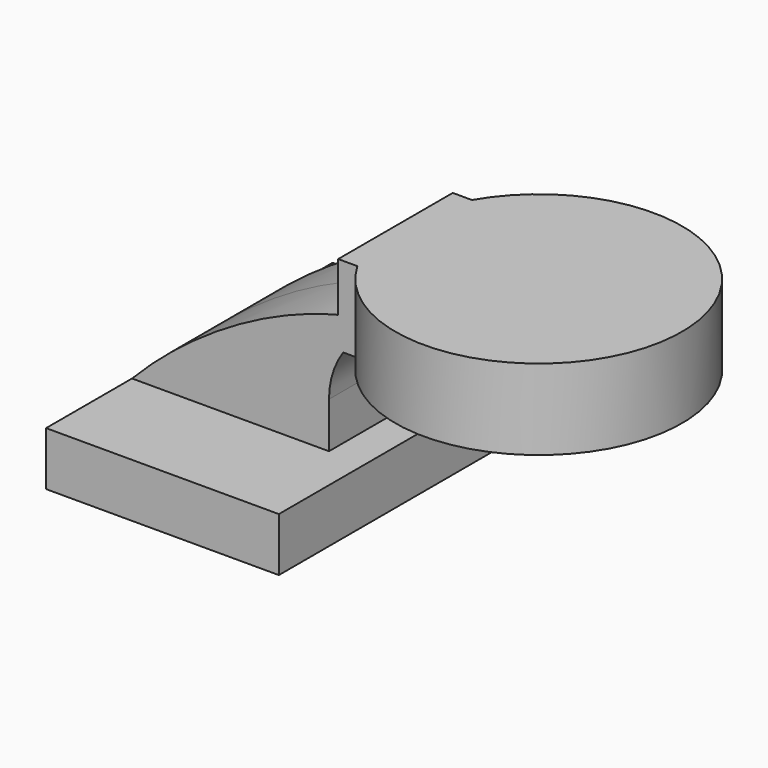
from build123d import *

# Parameters (mm, degrees)
F1_DEPTH = 63.5
F2_DEPTH = 25.4
F3_DEPTH = 25.4


# Not quite as in the source:
# - a feature names something its author has since deleted; it is built from what else it names


with BuildPart() as f1:
    # F0 (on Front) → F1 (new body, symmetric)
    with BuildSketch(Plane.XZ):
        Polygon((28.5749990565, 9.525), (-41.275, 9.525), (-41.275, -9.525), (41.275, -9.525), (41.275, 9.525), align=None)
    extrude(amount=F1_DEPTH, both=True)

    # F0 (on Front) → F2 (join, symmetric)
    with BuildSketch(Plane.XZ):
        with BuildLine():
            add(Edge.make_bspline(
                [(-41.275, 9.525), (-23.8584346144, 27.5869780948), (3.0069667421, 45.9865968148), (31.8262, 53.1677247911)],
                knots=[0, 0, 0, 0, 84.5177049164, 84.5177049164, 84.5177049164, 84.5177049164], degree=3))
            Line((-41.275, 9.525), (28.5749990565, 9.525))
            Line((28.5749990565, 9.525), (28.5749990565, 25.7647229111))
            ThreePointArc((28.5749990565, 25.7647229111), (29.8677699589, 34.2739896946), (33.6294204286, 42.0153631867))
            Line((33.6294204286, 42.0153631867), (31.8262, 42.0153631867))
            Line((31.8262, 42.0153631867), (31.8262, 53.1677247911))
        make_face()
    extrude(amount=F2_DEPTH, both=True)

    # F0 (on Front) → F3 (join, symmetric)
    with BuildSketch(Plane.XZ):
        Polygon((31.8262, 70.5903631867), (31.8262, 53.1677247911), (31.8262, 42.0153631867), (33.6294204286, 42.0153631867), (82.6262, 42.0153631867), (82.6262, 70.5903631867), align=None)
    extrude(amount=F3_DEPTH, both=True)

    # F0 (on Front) → F6 (revolve)
    with BuildSketch(Plane.XZ):
        Polygon((31.8262, 70.5903631867), (31.8262, 53.1677247911), (31.8262, 42.0153631867), (33.6294204286, 42.0153631867), (82.6262, 42.0153631867), (82.6262, 70.5903631867), align=None)
    revolve(axis=Axis((82.6262, 0, 56.3028631867), (0, 0, 1)))


solid = f1.part
